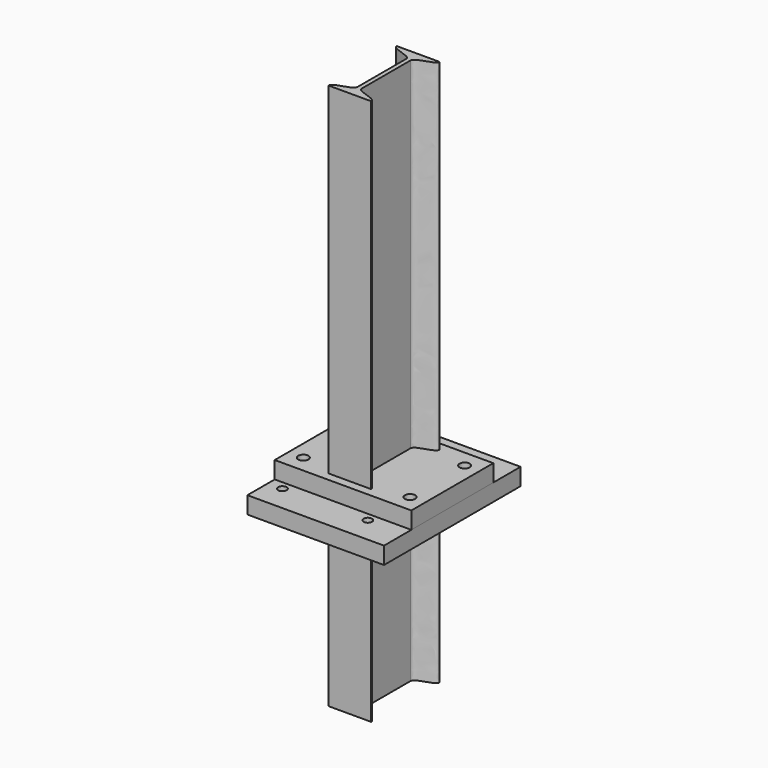
from build123d import *

# Parameters (mm, degrees)
F1_DEPTH = 420
F0_W     = 160
F0_H     = 120
F0_R     = 6
F2_DEPTH = 20
F3_DEPTH = 220
F4_W     = 160
F4_H     = 200
F4_R     = 5
F5_DEPTH = 20


with BuildPart() as f1:
    # F0 (on Top) → F1 (new body)
    with BuildSketch(Plane.XY):
        with BuildLine():
            Line((25, 50), (-25, 50))
            add(Edge.make_bspline(
                [(-25, 50), (-25, 43), (-2.5, 43), (-2.5, 35.375)],
                knots=[0, 0, 0, 0, 26.8354359942, 26.8354359942, 26.8354359942, 26.8354359942], degree=3))
            Line((-2.5, 35.375), (-2.5, -35.375))
            add(Edge.make_bspline(
                [(-25, -50), (-25, -43), (-2.5, -43), (-2.5, -35.375)],
                knots=[0, 0, 0, 0, 26.8354359942, 26.8354359942, 26.8354359942, 26.8354359942], degree=3))
            Line((-25, -50), (25, -50))
            add(Edge.make_bspline(
                [(25, -50), (25, -43), (2.5, -43), (2.5, -35.375)],
                knots=[0, 0, 0, 0, 26.8354359942, 26.8354359942, 26.8354359942, 26.8354359942], degree=3))
            Line((2.5, -35.375), (2.5, 35.375))
            add(Edge.make_bspline(
                [(2.5, 35.375), (2.5, 43), (25, 43), (25, 50)],
                knots=[0, 0, 0, 0, 26.8354359942, 26.8354359942, 26.8354359942, 26.8354359942], degree=3))
        make_face()
    extrude(amount=F1_DEPTH)

    # F0 (on Top) → F2 (join)
    with BuildSketch(Plane.XY):
        Rectangle(F0_W, F0_H)
        with Locations((-62.5, -40)):
            Circle(F0_R, mode=Mode.SUBTRACT)
        with Locations((62.5, -40)):
            Circle(F0_R, mode=Mode.SUBTRACT)
        with Locations((-62.5, 40)):
            Circle(F0_R, mode=Mode.SUBTRACT)
        with BuildLine():
            add(Edge.make_bspline(
                [(-25, 50), (-25, 43), (-2.5, 43), (-2.5, 35.375)],
                knots=[0, 0, 0, 0, 26.8354359942, 26.8354359942, 26.8354359942, 26.8354359942], degree=3))
            Line((-25, 50), (25, 50))
            add(Edge.make_bspline(
                [(2.5, 35.375), (2.5, 43), (25, 43), (25, 50)],
                knots=[0, 0, 0, 0, 26.8354359942, 26.8354359942, 26.8354359942, 26.8354359942], degree=3))
            Line((2.5, 35.375), (2.5, -35.375))
            add(Edge.make_bspline(
                [(25, -50), (25, -43), (2.5, -43), (2.5, -35.375)],
                knots=[0, 0, 0, 0, 26.8354359942, 26.8354359942, 26.8354359942, 26.8354359942], degree=3))
            Line((25, -50), (-25, -50))
            add(Edge.make_bspline(
                [(-25, -50), (-25, -43), (-2.5, -43), (-2.5, -35.375)],
                knots=[0, 0, 0, 0, 26.8354359942, 26.8354359942, 26.8354359942, 26.8354359942], degree=3))
            Line((-2.5, -35.375), (-2.5, 35.375))
        make_face(mode=Mode.SUBTRACT)
        with Locations((62.5, 40)):
            Circle(F0_R, mode=Mode.SUBTRACT)
        with BuildLine():
            Line((25, 50), (-25, 50))
            add(Edge.make_bspline(
                [(-25, 50), (-25, 43), (-2.5, 43), (-2.5, 35.375)],
                knots=[0, 0, 0, 0, 26.8354359942, 26.8354359942, 26.8354359942, 26.8354359942], degree=3))
            Line((-2.5, 35.375), (-2.5, -35.375))
            add(Edge.make_bspline(
                [(-25, -50), (-25, -43), (-2.5, -43), (-2.5, -35.375)],
                knots=[0, 0, 0, 0, 26.8354359942, 26.8354359942, 26.8354359942, 26.8354359942], degree=3))
            Line((-25, -50), (25, -50))
            add(Edge.make_bspline(
                [(25, -50), (25, -43), (2.5, -43), (2.5, -35.375)],
                knots=[0, 0, 0, 0, 26.8354359942, 26.8354359942, 26.8354359942, 26.8354359942], degree=3))
            Line((2.5, -35.375), (2.5, 35.375))
            add(Edge.make_bspline(
                [(2.5, 35.375), (2.5, 43), (25, 43), (25, 50)],
                knots=[0, 0, 0, 0, 26.8354359942, 26.8354359942, 26.8354359942, 26.8354359942], degree=3))
        make_face()
    extrude(amount=F2_DEPTH)


with BuildPart() as f3:
    # F0 (on Top) → F3 (new body)
    with BuildSketch(Plane.XY):
        with BuildLine():
            Line((25, 50), (-25, 50))
            add(Edge.make_bspline(
                [(-25, 50), (-25, 43), (-2.5, 43), (-2.5, 35.375)],
                knots=[0, 0, 0, 0, 26.8354359942, 26.8354359942, 26.8354359942, 26.8354359942], degree=3))
            Line((-2.5, 35.375), (-2.5, -35.375))
            add(Edge.make_bspline(
                [(-25, -50), (-25, -43), (-2.5, -43), (-2.5, -35.375)],
                knots=[0, 0, 0, 0, 26.8354359942, 26.8354359942, 26.8354359942, 26.8354359942], degree=3))
            Line((-25, -50), (25, -50))
            add(Edge.make_bspline(
                [(25, -50), (25, -43), (2.5, -43), (2.5, -35.375)],
                knots=[0, 0, 0, 0, 26.8354359942, 26.8354359942, 26.8354359942, 26.8354359942], degree=3))
            Line((2.5, -35.375), (2.5, 35.375))
            add(Edge.make_bspline(
                [(2.5, 35.375), (2.5, 43), (25, 43), (25, 50)],
                knots=[0, 0, 0, 0, 26.8354359942, 26.8354359942, 26.8354359942, 26.8354359942], degree=3))
        make_face()
    extrude(amount=-F3_DEPTH)

    # F4 (on Top) → F5 (join)
    with BuildSketch(Plane.XY):
        Rectangle(F4_W, F4_H)
        with Locations((-63, -70)):
            Circle(F4_R, mode=Mode.SUBTRACT)
        with Locations((37, -70)):
            Circle(F4_R, mode=Mode.SUBTRACT)
        with Locations((-63, 70)):
            Circle(F4_R, mode=Mode.SUBTRACT)
        with Locations((37, 70)):
            Circle(F4_R, mode=Mode.SUBTRACT)
    extrude(amount=-F5_DEPTH)


solid = Compound([f1.part, f3.part])
